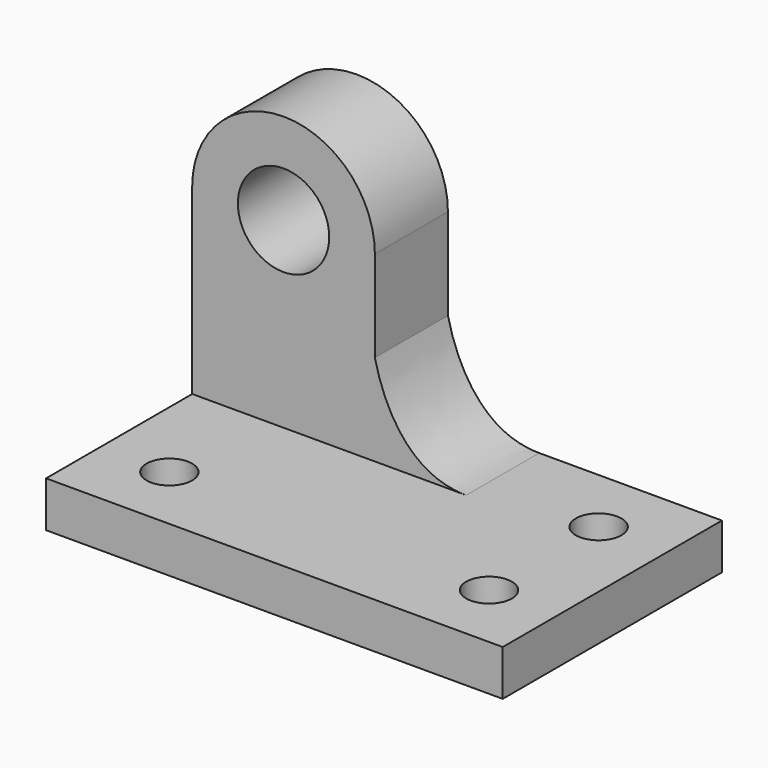
from build123d import *

# Parameters (mm, degrees)
F1_DEPTH = 12.7
F3_DEPTH = 25.4
F4_R     = 6.35
F5_DEPTH = 25.4
F6_R     = 3.175
F7_DEPTH = 25.4


with BuildPart() as f1:
    # F0 (on Front) → F1 (new body)
    with BuildSketch(Plane.XZ):
        with BuildLine():
            Line((-59.417062837, 42.575026238), (-59.417062837, 10.825026238))
            Line((-59.417062837, 10.825026238), (4.082937163, 10.825026238))
            Line((4.082937163, 10.825026238), (4.082937163, 17.175026238))
            Line((4.082937163, 17.175026238), (-21.317062837, 17.175026238))
            Line((-21.317062837, 17.175026238), (-34.017062837, 17.175026238))
            Line((-34.017062837, 17.175026238), (-34.017062837, 29.875026238))
            add(Edge.make_bspline(
                [(-34.017062837, 42.575026238), (-34.6135151064, 38.5440672107), (-35.1151608476, 34.6686954927), (-34.017062837, 29.875026238)],
                knots=[0, 0, 0, 0, 0.4567863831, 0.4567863831, 0.4567863831, 0.4567863831], degree=3))
            Line((-34.017062837, 42.575026238), (-59.417062837, 42.575026238))
        make_face()
        with BuildLine():
            ThreePointArc((-34.017062837, 42.575026238), (-46.717062837, 55.275026238), (-59.417062837, 42.575026238))
            Line((-59.417062837, 42.575026238), (-34.017062837, 42.575026238))
        make_face()
        with BuildLine():
            Line((-34.017062837, 29.875026238), (-34.017062837, 42.575026238))
            add(Edge.make_bspline(
                [(-34.017062837, 42.575026238), (-34.6135151064, 38.5440672107), (-35.1151608476, 34.6686954927), (-34.017062837, 29.875026238)],
                knots=[0, 0, 0, 0, 0.4567863831, 0.4567863831, 0.4567863831, 0.4567863831], degree=3))
        make_face()
        with BuildLine():
            Line((-34.017062837, 17.175026238), (-21.317062837, 17.175026238))
            add(Edge.make_bspline(
                [(-34.017062837, 29.875026238), (-32.7111968699, 24.1743606533), (-29.1429515928, 17.175026238), (-21.317062837, 17.175026238)],
                knots=[0.4567863831, 0.4567863831, 0.4567863831, 0.4567863831, 1, 1, 1, 1], degree=3))
            Line((-34.017062837, 29.875026238), (-34.017062837, 17.175026238))
        make_face()
    extrude(amount=F1_DEPTH)

    # F2 (on face) → F3 (join)
    with BuildSketch(Plane.XZ.offset(12.7)):
        Polygon((4.082937163, 17.175026238), (-21.317062837, 17.175026238), (-59.417062837, 17.175026238), (-59.417062837, 10.825026238), (4.082937163, 10.825026238), align=None)
    extrude(amount=F3_DEPTH)

    # F4 (on face) → F5 (cut)
    with BuildSketch(Plane.XZ.offset(12.7)):
        with Locations((-46.717062837, 42.575026238)):
            Circle(F4_R)
    extrude(amount=-F5_DEPTH, mode=Mode.SUBTRACT)

    # F6 (on face) → F7 (cut)
    with BuildSketch(Plane.XY.offset(17.175026238)):
        with Locations((-49.892062837, -28.575)):
            Circle(F6_R)
        with Locations((-5.442062837, -28.575)):
            Circle(F6_R)
        with Locations((-5.442062837, -9.525)):
            Circle(F6_R)
    extrude(amount=-F7_DEPTH, mode=Mode.SUBTRACT)


solid = f1.part
